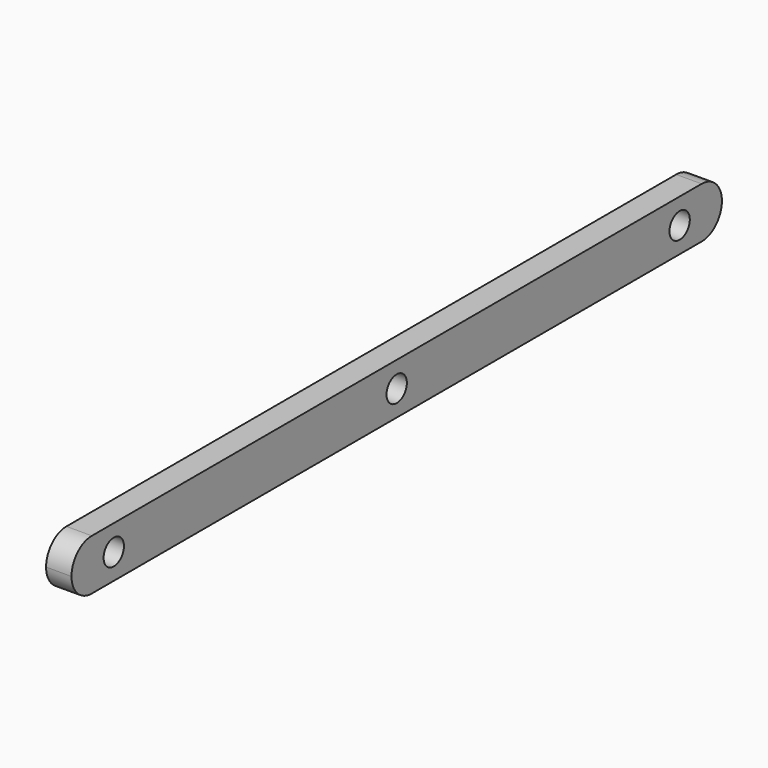
from build123d import *

# Parameters (mm, degrees)
F0_W     = 101.6
F0_H     = 6.35
F0_R     = 1.5875
F1_DEPTH = 3.175
F2_R     = 3.17499
F3_R     = 3.17499


# Not quite as in the source:
# - a fillet or chamfer is up to 0.001 mm smaller than in the source, because OpenCascade refuses the exact size


with BuildPart() as f1:
    # F0 (on Right) → F1 (new body)
    with BuildSketch(Plane.YZ):
        with Locations((50.8, -3.175)):
            Rectangle(F0_W, F0_H)
        with Locations((6.604, -3.175)):
            Circle(F0_R, mode=Mode.SUBTRACT)
        with Locations((50.8, -3.175)):
            Circle(F0_R, mode=Mode.SUBTRACT)
        with Locations((94.996, -3.175)):
            Circle(F0_R, mode=Mode.SUBTRACT)
    extrude(amount=F1_DEPTH)

    # F2 (radius 3.175 in the source; OpenCascade refuses exactly that, so slightly less here)
    f2_edges = [f1.edges().sort_by_distance(p)[0] for p in [
        (1.5875, 0, 0),
        (1.5875, 0, -6.35),
    ]]
    fillet(f2_edges, radius=F2_R)

    # F3 (radius 3.175 in the source; OpenCascade refuses exactly that, so slightly less here)
    f3_edges = [f1.edges().sort_by_distance(p)[0] for p in [
        (1.5875, 101.6, 0),
        (1.5875, 101.6, -6.35),
    ]]
    fillet(f3_edges, radius=F3_R)


solid = f1.part
